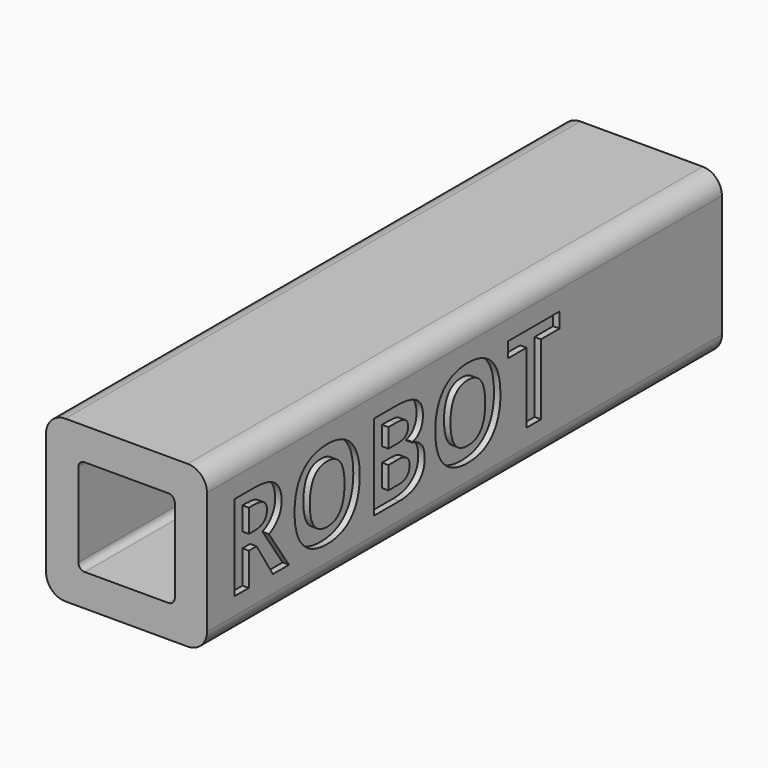
from build123d import *

# Parameters (mm, degrees)
F0_W         = 25
F0_H         = 25
F0_W_2       = 15
F0_H_2       = 15
F1_DEPTH     = 100
F2_R         = 1
F3_R         = 3
F4_TEXT_SIZE = 18.617022498
F5_DEPTH     = 1


# Not quite as in the source:
# - Text() gives the source's letters only with a copy of the font that has no kerning and outlines rounded to 1/6400 em; it was checked with that copy


with BuildPart() as f1:
    # F0 (on Front) → F1 (new body)
    with BuildSketch(Plane.XZ):
        Rectangle(F0_W, F0_H)
        Rectangle(F0_W_2, F0_H_2, mode=Mode.SUBTRACT)
    extrude(amount=F1_DEPTH)

    # F2
    f2_edges = [f1.edges().sort_by_distance(p)[0] for p in [
        (-7.5, -50, 7.5),
        (7.5, -50, 7.5),
        (7.5, -50, -7.5),
        (-7.5, -50, -7.5),
    ]]
    fillet(f2_edges, radius=F2_R)

    # F3
    f3_edges = [f1.edges().sort_by_distance(p)[0] for p in [
        (12.5, -50, 12.5),
        (-12.5, -50, 12.5),
        (-12.5, -50, -12.5),
        (12.5, -50, -12.5),
    ]]
    fillet(f3_edges, radius=F3_R)

    # F4 (on face) → F5 (cut)
    with BuildSketch(Plane.YZ.offset(12.5)):
        with Locations((-96.3655412197, -6.8119987845)):
            Text('ROBOT', F4_TEXT_SIZE, font='Open Sans', font_style=FontStyle.BOLD, text_align=(TextAlign.LEFT, TextAlign.BOTTOM))
    extrude(amount=-F5_DEPTH, mode=Mode.SUBTRACT)


solid = f1.part
